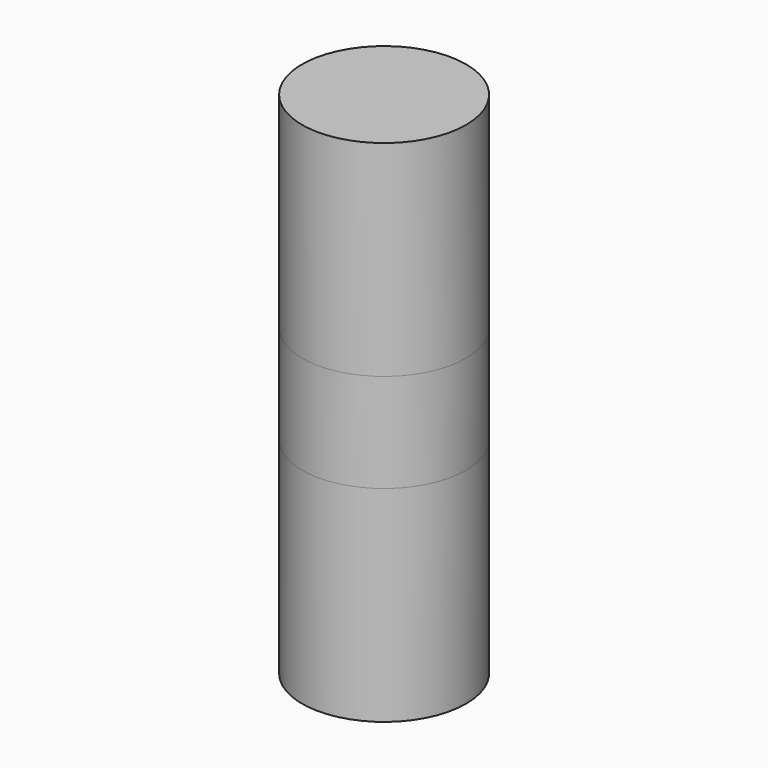
from build123d import *

# Parameters (mm, degrees)
F0_R      = 10.1411241646
F1_DEPTH  = 25.4
F1_FACE_R = 10.1411241646
F2_DEPTH  = 37.6


# Not quite as in the source:
# - a feature names something its author has since deleted; it is built from what else it names


with BuildPart() as f1:
    # F0 (on Top) → F1 (new body)
    with BuildSketch(Plane.XY):
        Circle(F0_R)
    extrude(amount=F1_DEPTH)

    # F0 (on Top) + F1_face (on face) → F2 (join)
    with BuildSketch(Plane.XY):
        Circle(F0_R)
    with BuildSketch(Plane.XY.offset(25.4)):
        Circle(F1_FACE_R)
    extrude(amount=-F2_DEPTH)


solid = f1.part
